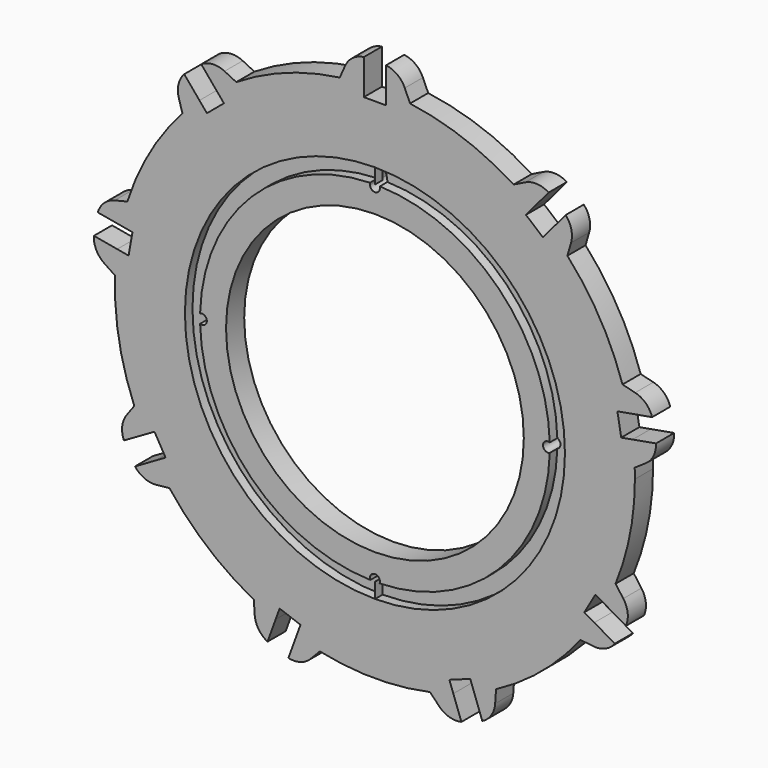
from build123d import *

# Parameters (mm, degrees)
F0_R     = 1.3335
F0_R_2   = 40.005
F1_DEPTH = 6.096
F2_R     = 51.054
F3_DEPTH = 2.54
F5_DEPTH = 2.54


# Not quite as in the source:
# - a pattern or mirror of a feature is missing from the dataset's text; its kind, count and spacing are read off the source's solid


with BuildPart() as f1:
    # F0 (on Front) → F1 (new body)
    with BuildSketch(Plane.XZ):
        with BuildLine():
            ThreePointArc((64.6559292996, -26.4316724103), (68.5391828138, -13.4685900974), (69.85, 0))
            ThreePointArc((69.85, 0), (69.8367147463, 1.3622677557), (69.796864039, 2.7240173131))
            ThreePointArc((69.796864039, 2.7240173131), (69.5954392681, 5.9579638364), (69.2442547313, 9.179089645))
            Line((69.2442547313, 9.179089645), (66.1803099183, 8.6388335071))
            Line((66.1803099183, 8.6388335071), (65.1438039458, 14.5171509848))
            Line((65.1438039458, 14.5171509848), (68.2077487588, 15.0574071227))
            ThreePointArc((68.2077487588, 15.0574071227), (67.4360643659, 18.2043874613), (66.5192668833, 21.3121944743))
            ThreePointArc((66.5192668833, 21.3121944743), (60.4918744543, 34.925), (51.7165352668, 46.9512777249))
            ThreePointArc((51.7165352668, 46.9512777249), (49.4834941848, 49.2991511414), (47.1439714628, 51.5409395987))
            Line((47.1439714628, 51.5409395987), (45.1441235163, 49.1576136238))
            Line((45.1441235163, 49.1576136238), (40.5716042354, 52.9944128661))
            Line((40.5716042354, 52.9944128661), (42.5714521818, 55.3777388409))
            ThreePointArc((42.5714521818, 55.3777388409), (39.9574676712, 57.2924364755), (37.257500213, 59.0838487057))
            ThreePointArc((37.257500213, 59.0838487057), (23.8901070113, 65.6375295619), (9.4374648779, 69.2095134839))
            ThreePointArc((9.4374648779, 69.2095134839), (6.2176722246, 69.5727177283), (2.9845, 69.7862111004))
            Line((2.9845, 69.7862111004), (2.9845, 66.675))
            Line((2.9845, 66.675), (-2.9845, 66.675))
            Line((-2.9845, 66.675), (-2.9845, 69.7862111004))
            ThreePointArc((-2.9845, 69.7862111004), (-6.2176722246, 69.5727177283), (-9.4374648779, 69.2095134839))
            ThreePointArc((-9.4374648779, 69.2095134839), (-23.8901070113, 65.6375295619), (-37.257500213, 59.0838487057))
            ThreePointArc((-37.257500213, 59.0838487057), (-39.9574676712, 57.2924364755), (-42.5714521818, 55.3777388409))
            Line((-42.5714521818, 55.3777388409), (-40.5716042354, 52.9944128661))
            Line((-40.5716042354, 52.9944128661), (-45.1441235163, 49.1576136238))
            Line((-45.1441235163, 49.1576136238), (-47.1439714628, 51.5409395987))
            ThreePointArc((-47.1439714628, 51.5409395987), (-49.4834941848, 49.2991511414), (-51.7165352668, 46.9512777249))
            ThreePointArc((-51.7165352668, 46.9512777249), (-60.4918744543, 34.925), (-66.5192668833, 21.3121944743))
            ThreePointArc((-66.5192668833, 21.3121944743), (-67.4360643659, 18.2043874613), (-68.2077487588, 15.0574071227))
            Line((-68.2077487588, 15.0574071227), (-65.1438039458, 14.5171509848))
            Line((-65.1438039458, 14.5171509848), (-66.1803099183, 8.6388335071))
            Line((-66.1803099183, 8.6388335071), (-69.2442547313, 9.179089645))
            ThreePointArc((-69.2442547313, 9.179089645), (-69.5954392681, 5.9579638364), (-69.796864039, 2.7240173131))
            ThreePointArc((-69.796864039, 2.7240173131), (-68.7888215479, -12.12932521), (-64.6559292996, -26.4316724103))
            ThreePointArc((-64.6559292996, -26.4316724103), (-63.3605770754, -29.4016967653), (-61.9288816468, -32.3084527326))
            Line((-61.9288816468, -32.3084527326), (-59.2344937973, -30.7528471824))
            Line((-59.2344937973, -30.7528471824), (-56.2499937973, -35.9221528176))
            Line((-56.2499937973, -35.9221528176), (-58.9443816468, -37.4777583678))
            ThreePointArc((-58.9443816468, -37.4777583678), (-57.1429048508, -40.1710209631), (-55.2184644216, -42.7778410736))
            ThreePointArc((-55.2184644216, -42.7778410736), (-44.8987145366, -53.5082043519), (-32.539363826, -61.8078660188))
            ThreePointArc((-32.539363826, -61.8078660188), (-29.6379715969, -63.2504003119), (-26.6728025495, -64.5568284859))
            Line((-26.6728025495, -64.5568284859), (-25.608705683, -61.6332463731))
            Line((-25.608705683, -61.6332463731), (-19.9996804295, -63.6747646087))
            Line((-19.9996804295, -63.6747646087), (-21.063777296, -66.5983467214))
            ThreePointArc((-21.063777296, -66.5983467214), (-17.9525701811, -67.5035386028), (-14.8027316165, -68.2634721992))
            ThreePointArc((-14.8027316165, -68.2634721992), (0, -69.85), (14.8027316165, -68.2634721992))
            ThreePointArc((14.8027316165, -68.2634721992), (17.9525701811, -67.5035386028), (21.063777296, -66.5983467214))
            Line((21.063777296, -66.5983467214), (19.9996804295, -63.6747646087))
            Line((19.9996804295, -63.6747646087), (25.608705683, -61.6332463731))
            Line((25.608705683, -61.6332463731), (26.6728025495, -64.5568284859))
            ThreePointArc((26.6728025495, -64.5568284859), (29.6379715969, -63.2504003119), (32.539363826, -61.8078660188))
            ThreePointArc((32.539363826, -61.8078660188), (44.8987145366, -53.5082043519), (55.2184644216, -42.7778410736))
            ThreePointArc((55.2184644216, -42.7778410736), (57.1429048508, -40.1710209631), (58.9443816468, -37.4777583678))
            Line((58.9443816468, -37.4777583678), (56.2499937973, -35.9221528176))
            Line((56.2499937973, -35.9221528176), (59.2344937973, -30.7528471824))
            Line((59.2344937973, -30.7528471824), (61.9288816468, -32.3084527326))
            ThreePointArc((61.9288816468, -32.3084527326), (63.3605770754, -29.4016967653), (64.6559292996, -26.4316724103))
        make_face()
        with Locations((0, -46.4947)):
            Circle(F0_R, mode=Mode.SUBTRACT)
        with Locations((-46.4947, 0)):
            Circle(F0_R, mode=Mode.SUBTRACT)
        Circle(F0_R_2, mode=Mode.SUBTRACT)
        with Locations((46.4947, 0)):
            Circle(F0_R, mode=Mode.SUBTRACT)
        with BuildLine():
            ThreePointArc((1.3333628788, 46.4755771511), (0, 45.1612), (-1.3333628788, 46.4755771511))
            ThreePointArc((-1.3333628788, 46.4755771511), (-1.0083284803, 48.7431296807), (0, 50.8))
            ThreePointArc((0, 50.8), (1.0083284803, 48.7431296807), (1.3333628788, 46.4755771511))
        make_face(mode=Mode.SUBTRACT)
        with BuildLine():
            ThreePointArc((-42.5714521818, 55.3777388409), (-39.9574676712, 57.2924364755), (-37.257500213, 59.0838487057))
            Line((-37.257500213, 59.0838487057), (-40.4029688253, 60.6296034594))
            ThreePointArc((-40.4029688253, 60.6296034594), (-43.5829240562, 61.2692328974), (-46.6639038364, 60.2549328028))
            Line((-46.6639038364, 60.2549328028), (-42.5714521818, 55.3777388409))
        make_face()
        with BuildLine():
            ThreePointArc((-51.7165352668, 46.9512777249), (-49.4834941848, 49.2991511414), (-47.1439714628, 51.5409395987))
            Line((-47.1439714628, 51.5409395987), (-51.2364231174, 56.4181335606))
            ThreePointArc((-51.2364231174, 56.4181335606), (-52.7703202388, 53.5600921491), (-52.69260164, 50.3173770972))
            Line((-52.69260164, 50.3173770972), (-51.7165352668, 46.9512777249))
        make_face()
        with BuildLine():
            ThreePointArc((-9.4374648779, 69.2095134839), (-6.2176722246, 69.5727177283), (-2.9845, 69.7862111004))
            Line((-2.9845, 69.7862111004), (-2.9845, 76.1529356498))
            ThreePointArc((-2.9845, 76.1529356498), (-5.9966469734, 74.9495189725), (-8.0214881298, 72.415498574))
            Line((-8.0214881298, 72.415498574), (-9.4374648779, 69.2095134839))
        make_face()
        with BuildLine():
            ThreePointArc((2.9845, 69.7862111004), (6.2176722246, 69.5727177283), (9.4374648779, 69.2095134839))
            Line((9.4374648779, 69.2095134839), (8.0214881298, 72.415498574))
            ThreePointArc((8.0214881298, 72.415498574), (5.9966469734, 74.9495189725), (2.9845, 76.1529356498))
            Line((2.9845, 76.1529356498), (2.9845, 69.7862111004))
        make_face()
        with BuildLine():
            ThreePointArc((37.257500213, 59.0838487057), (39.9574676712, 57.2924364755), (42.5714521818, 55.3777388409))
            Line((42.5714521818, 55.3777388409), (46.6639038364, 60.2549328028))
            ThreePointArc((46.6639038364, 60.2549328028), (43.5829240562, 61.2692328974), (40.4029688253, 60.6296034594))
            Line((40.4029688253, 60.6296034594), (37.257500213, 59.0838487057))
        make_face()
        with BuildLine():
            ThreePointArc((47.1439714628, 51.5409395987), (49.4834941848, 49.2991511414), (51.7165352668, 46.9512777249))
            Line((51.7165352668, 46.9512777249), (52.69260164, 50.3173770972))
            ThreePointArc((52.69260164, 50.3173770972), (52.7703202388, 53.5600921491), (51.2364231174, 56.4181335606))
            Line((51.2364231174, 56.4181335606), (47.1439714628, 51.5409395987))
        make_face()
        with BuildLine():
            ThreePointArc((66.5192668833, 21.3121944743), (67.4360643659, 18.2043874613), (68.2077487588, 15.0574071227))
            Line((68.2077487588, 15.0574071227), (74.4777484563, 16.1629772384))
            ThreePointArc((74.4777484563, 16.1629772384), (72.7695605496, 18.920391818), (69.922427638, 20.4744430631))
            Line((69.922427638, 20.4744430631), (66.5192668833, 21.3121944743))
        make_face()
        with BuildLine():
            ThreePointArc((69.2442547313, 9.179089645), (69.5954392681, 5.9579638364), (69.796864039, 2.7240173131))
            Line((69.796864039, 2.7240173131), (72.7082612299, 4.6751956613))
            ThreePointArc((72.7082612299, 4.6751956613), (74.8521741876, 7.1093029551), (75.5142544288, 10.2846597607))
            Line((75.5142544288, 10.2846597607), (69.2442547313, 9.179089645))
        make_face()
        with BuildLine():
            Line((66.7244054577, -29.2609367904), (64.6559292996, -26.4316724103))
            ThreePointArc((64.6559292996, -26.4316724103), (63.3605770754, -29.4016967653), (61.9288816468, -32.3084527326))
            Line((61.9288816468, -32.3084527326), (67.4426268455, -35.4918150073))
            ThreePointArc((67.4426268455, -35.4918150073), (67.9065109183, -32.2815108698), (66.7244054577, -29.2609367904))
        make_face()
        with BuildLine():
            Line((64.4581268455, -40.6611206425), (58.9443816468, -37.4777583678))
            ThreePointArc((58.9443816468, -37.4777583678), (57.1429048508, -40.1710209631), (55.2184644216, -42.7778410736))
            Line((55.2184644216, -42.7778410736), (58.7029173279, -43.1545617836))
            ThreePointArc((58.7029173279, -43.1545617836), (61.9098639449, -42.6680081027), (64.4581268455, -40.6611206425))
        make_face()
        with BuildLine():
            Line((23.2413253389, -72.581110799), (21.063777296, -66.5983467214))
            ThreePointArc((21.063777296, -66.5983467214), (17.9525701811, -67.5035386028), (14.8027316165, -68.2634721992))
            Line((14.8027316165, -68.2634721992), (17.229825998, -70.7918201604))
            ThreePointArc((17.229825998, -70.7918201604), (19.9992403108, -72.4804839672), (23.2413253389, -72.581110799))
        make_face()
        with BuildLine():
            Line((32.3052924046, -65.3047991207), (32.539363826, -61.8078660188))
            ThreePointArc((32.539363826, -61.8078660188), (29.6379715969, -63.2504003119), (26.6728025495, -64.5568284859))
            Line((26.6728025495, -64.5568284859), (28.8503505923, -70.5395925635))
            ThreePointArc((28.8503505923, -70.5395925635), (31.2692501315, -68.3785358526), (32.3052924046, -65.3047991207))
        make_face()
        with BuildLine():
            Line((-28.8503505923, -70.5395925635), (-26.6728025495, -64.5568284859))
            ThreePointArc((-26.6728025495, -64.5568284859), (-29.6379715969, -63.2504003119), (-32.539363826, -61.8078660188))
            Line((-32.539363826, -61.8078660188), (-32.3052924046, -65.3047991207))
            ThreePointArc((-32.3052924046, -65.3047991207), (-31.2692501315, -68.3785358526), (-28.8503505923, -70.5395925635))
        make_face()
        with BuildLine():
            Line((-17.229825998, -70.7918201604), (-14.8027316165, -68.2634721992))
            ThreePointArc((-14.8027316165, -68.2634721992), (-17.9525701811, -67.5035386028), (-21.063777296, -66.5983467214))
            Line((-21.063777296, -66.5983467214), (-23.2413253389, -72.581110799))
            ThreePointArc((-23.2413253389, -72.581110799), (-19.9992403108, -72.4804839672), (-17.229825998, -70.7918201604))
        make_face()
        with BuildLine():
            Line((-58.7029173279, -43.1545617836), (-55.2184644216, -42.7778410736))
            ThreePointArc((-55.2184644216, -42.7778410736), (-57.1429048508, -40.1710209631), (-58.9443816468, -37.4777583678))
            Line((-58.9443816468, -37.4777583678), (-64.4581268455, -40.6611206425))
            ThreePointArc((-64.4581268455, -40.6611206425), (-61.9098639449, -42.6680081027), (-58.7029173279, -43.1545617836))
        make_face()
        with BuildLine():
            Line((-67.4426268455, -35.4918150073), (-61.9288816468, -32.3084527326))
            ThreePointArc((-61.9288816468, -32.3084527326), (-63.3605770754, -29.4016967653), (-64.6559292996, -26.4316724103))
            Line((-64.6559292996, -26.4316724103), (-66.7244054577, -29.2609367904))
            ThreePointArc((-66.7244054577, -29.2609367904), (-67.9065109183, -32.2815108698), (-67.4426268455, -35.4918150073))
        make_face()
        with BuildLine():
            Line((-72.7082612299, 4.6751956613), (-69.796864039, 2.7240173131))
            ThreePointArc((-69.796864039, 2.7240173131), (-69.5954392681, 5.9579638364), (-69.2442547313, 9.179089645))
            Line((-69.2442547313, 9.179089645), (-75.5142544288, 10.2846597607))
            ThreePointArc((-75.5142544288, 10.2846597607), (-74.8521741876, 7.1093029551), (-72.7082612299, 4.6751956613))
        make_face()
        with BuildLine():
            ThreePointArc((-68.2077487588, 15.0574071227), (-67.4360643659, 18.2043874613), (-66.5192668833, 21.3121944743))
            Line((-66.5192668833, 21.3121944743), (-69.922427638, 20.4744430631))
            ThreePointArc((-69.922427638, 20.4744430631), (-72.7695605496, 18.920391818), (-74.4777484563, 16.1629772384))
            Line((-74.4777484563, 16.1629772384), (-68.2077487588, 15.0574071227))
        make_face()
    extrude(amount=F1_DEPTH)

    # F2 (on face) → F3 (cut)
    with BuildSketch(Plane.XZ.offset(6.096)):
        Circle(F2_R)
        with BuildLine():
            ThreePointArc((1.3237188184, 46.9713515719), (33.2549291255, 33.1989425865), (46.9735153237, 1.2445714667))
            ThreePointArc((46.9735153237, 1.2445714667), (47.5939548576, 0.7548913882), (47.8282, 0))
            ThreePointArc((47.8282, 0), (47.5939548576, -0.7548913882), (46.9735153237, -1.2445714667))
            ThreePointArc((46.9735153237, -1.2445714667), (33.226947648, -33.226947648), (1.2445714667, -46.9735153237))
            ThreePointArc((1.2445714667, -46.9735153237), (0, -47.8282), (-1.2445714667, -46.9735153237))
            ThreePointArc((-1.2445714667, -46.9735153237), (-33.226947648, -33.226947648), (-46.9735153237, -1.2445714667))
            ThreePointArc((-46.9735153237, -1.2445714667), (-47.8282, 0), (-46.9735153237, 1.2445714667))
            ThreePointArc((-46.9735153237, 1.2445714667), (-33.2549291255, 33.1989425865), (-1.3237188184, 46.9713515719))
            ThreePointArc((-1.3237188184, 46.9713515719), (-0.9312725034, 48.9788228036), (0, 50.8))
            ThreePointArc((0, 50.8), (0.9312725034, 48.9788228036), (1.3237188184, 46.9713515719))
        make_face(mode=Mode.SUBTRACT)
    extrude(amount=-F3_DEPTH, mode=Mode.SUBTRACT)

    # F4 (on face) → F5 (join, through all)
    with BuildSketch(Plane.XZ.offset(6.096)):
        with BuildLine():
            ThreePointArc((0.0254, 51.0539936816), (0, 51.054), (-0.0254, 51.0539936816))
            Line((-0.0254, 51.0539936816), (-0.0254, 46.9899931351))
            ThreePointArc((-0.0254, 46.9899931351), (0, 46.99), (0.0254, 46.9899931351))
            Line((0.0254, 46.9899931351), (0.0254, 51.0539936816))
        make_face()
    f5 = extrude(amount=-F5_DEPTH)

    # F5_copies: F5 across plane
    add(f5.mirror(Plane(origin=(0, 0, 0), x_dir=(-1, 0, 0), z_dir=(0, 0, -1))))


solid = f1.part
